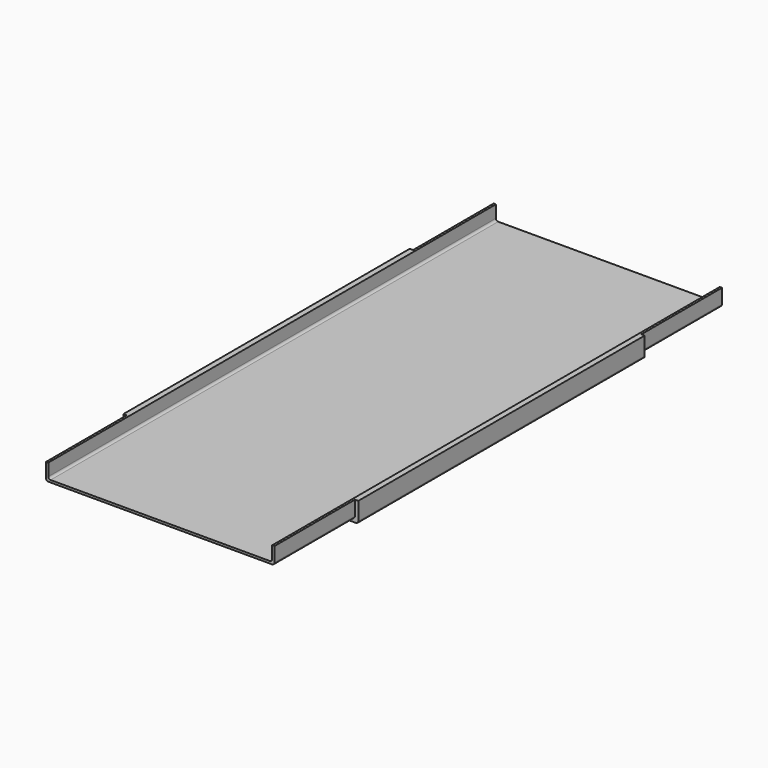
from build123d import *

# Parameters (mm, degrees)
F1_DEPTH = 500
F2_DEPTH = 90


# Not quite as in the source:
# - a pattern or mirror of a feature is missing from the dataset's text; its kind, count and spacing are read off the source's solid


with BuildPart() as f1:
    # F0 (on Front) → F1 (new body)
    with BuildSketch(Plane.XZ):
        with BuildLine():
            Line((102, 0), (100, 0))
            Line((100, 0), (100, -11))
            ThreePointArc((100, -11), (99.4142135624, -12.4142135624), (98, -13))
            Line((98, -13), (0, -13))
            Line((0, -13), (-98, -13))
            ThreePointArc((-98, -13), (-99.4142135624, -12.4142135624), (-100, -11))
            Line((-100, -11), (-100, 0))
            Line((-100, 0), (-102, 0))
            Line((-102, 0), (-102, -13))
            ThreePointArc((-102, -13), (-101.4142135624, -14.4142135624), (-100, -15))
            Line((-100, -15), (100, -15))
            ThreePointArc((100, -15), (101.4142135624, -14.4142135624), (102, -13))
            Line((102, -13), (102, 0))
        make_face()
        with BuildLine():
            Line((105, 0), (102, 0))
            Line((102, 0), (102, -13))
            ThreePointArc((102, -13), (101.4142135624, -14.4142135624), (100, -15))
            Line((100, -15), (-100, -15))
            ThreePointArc((-100, -15), (-101.4142135624, -14.4142135624), (-102, -13))
            Line((-102, -13), (-102, 0))
            Line((-102, 0), (-105, 0))
            Line((-105, 0), (-105, -16))
            ThreePointArc((-105, -16), (-104.4142135624, -17.4142135624), (-103, -18))
            Line((-103, -18), (0, -18))
            Line((0, -18), (103, -18))
            ThreePointArc((103, -18), (104.4142135624, -17.4142135624), (105, -16))
            Line((105, -16), (105, 0))
        make_face()
    extrude(amount=F1_DEPTH)

    # F0 (on Front) → F2 (cut)
    with BuildSketch(Plane.XZ):
        with BuildLine():
            Line((105, 0), (102, 0))
            Line((102, 0), (102, -13))
            ThreePointArc((102, -13), (101.4142135624, -14.4142135624), (100, -15))
            Line((100, -15), (-100, -15))
            ThreePointArc((-100, -15), (-101.4142135624, -14.4142135624), (-102, -13))
            Line((-102, -13), (-102, 0))
            Line((-102, 0), (-105, 0))
            Line((-105, 0), (-105, -16))
            ThreePointArc((-105, -16), (-104.4142135624, -17.4142135624), (-103, -18))
            Line((-103, -18), (0, -18))
            Line((0, -18), (103, -18))
            ThreePointArc((103, -18), (104.4142135624, -17.4142135624), (105, -16))
            Line((105, -16), (105, 0))
        make_face()
    f2 = extrude(amount=F2_DEPTH, mode=Mode.SUBTRACT)

    # F2_copies: F2 across plane
    add(f2.mirror(Plane(origin=(0, -250, 0), x_dir=(0, 0, -1), z_dir=(0, -1, 0))), mode=Mode.SUBTRACT)


solid = f1.part
